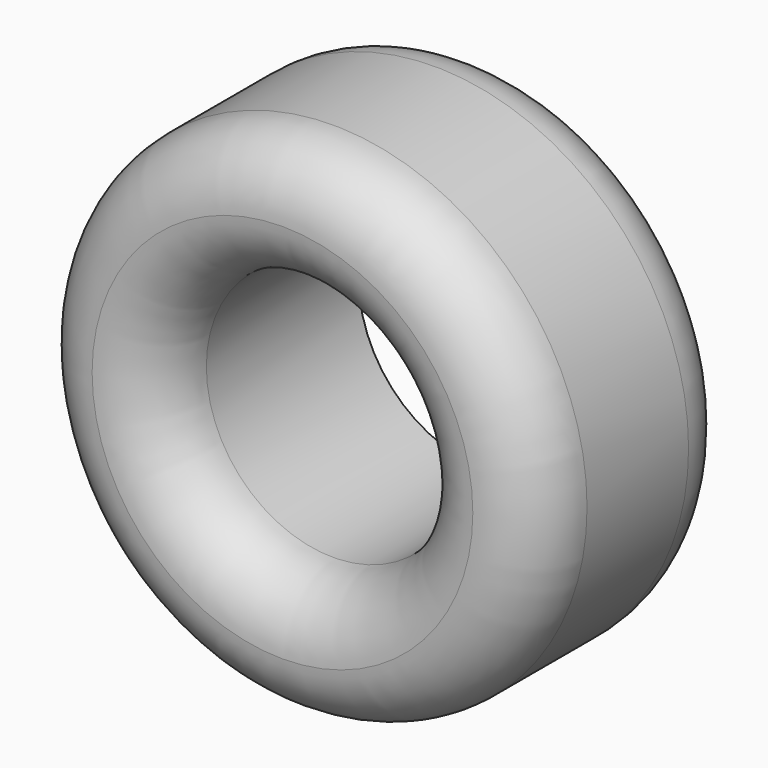
from build123d import *

# Parameters (mm, degrees)
F3_R     = 25.4
F4_DEPTH = 25.4
F6_D     = 25.4
F7_R     = 6.34999
F8_R     = 6.35


# Not quite as in the source:
# - a fillet or chamfer is up to 0.001 mm smaller than in the source, because OpenCascade refuses the exact size
# - the program builds the solid bodies; features that only make, move or delete a surface that nothing else refers to are left out


with BuildPart() as f4:
    # F3 (on Front) → F4 (new body)
    with BuildSketch(Plane.XZ):
        Circle(F3_R)
    extrude(amount=F4_DEPTH)

    # F6 (through all)
    with Locations(Plane.XZ.offset(25.4)):
        with Locations((0, 0)):
            Hole(F6_D / 2)

    # F7 (radius 6.35 in the source; OpenCascade refuses exactly that, so slightly less here)
    f7_edges = [f4.edges().sort_by_distance(p)[0] for p in [
        (-25.4, -25.4, 0),
        (-12.7, -25.4, 0),
    ]]
    fillet(f7_edges, radius=F7_R)

    # F8
    f8_edges = [f4.edges().sort_by_distance(p)[0] for p in [
        (-25.4, 0, 0),
    ]]
    fillet(f8_edges, radius=F8_R)


solid = f4.part
